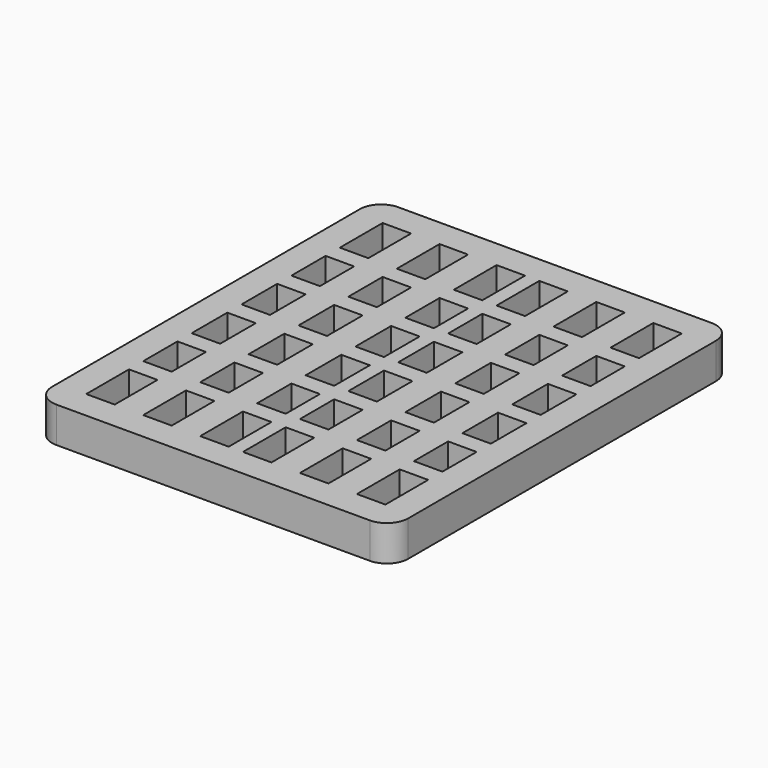
from build123d import *

# Parameters (mm, degrees)
F1_DEPTH = 5
F0_W     = 4
F0_H     = 7.5
F0_H_2   = 6.25
F0_H_3   = 6
F0_W_2   = 2
F0_H_4   = 2.5
F2_DEPTH = 5


# Not quite as in the source:
# - a feature names something its author has since deleted; it is built from what else it names


with BuildPart() as f1:
    # F0 (on Top) → F1 (new body)
    with BuildSketch(Plane.XY):
        with BuildLine():
            ThreePointArc((0, 3), (0.8786796564, 0.8786796564), (3, 0))
            Line((3, 0), (47, 0))
            ThreePointArc((47, 0), (49.1213203436, 0.8786796564), (50, 3))
            Line((50, 3), (50, 57))
            ThreePointArc((50, 57), (49.1213203436, 59.1213203436), (47, 60))
            Line((47, 60), (25, 60))
            Line((25, 60), (3, 60))
            ThreePointArc((3, 60), (0.8786796564, 59.1213203436), (0, 57))
            Line((0, 57), (0, 3))
        make_face()
        Polygon((24, 56), (25, 56), (26, 56), (30, 56), (34, 56), (38, 56), (42, 56), (46, 56), (46, 48.5), (46, 46), (46, 40), (46, 37.5), (46, 31.25), (46, 28.75), (46, 22.5), (46, 20), (46, 14), (46, 11.5), (46, 4), (42, 4), (38, 4), (34, 4), (30, 4), (26, 4), (24, 4), (20, 4), (16, 4), (12, 4), (8, 4), (4, 4), (4, 11.5), (4, 14), (4, 20), (4, 22.5), (4, 28.75), (4, 31.25), (4, 37.5), (4, 40), (4, 46), (4, 48.5), (4, 56), (8, 56), (12, 56), (16, 56), (20, 56), align=None, mode=Mode.SUBTRACT)
    extrude(amount=F1_DEPTH)

    # F0 (on Top) → F2 (join)
    with BuildSketch(Plane.XY):
        with BuildLine():
            ThreePointArc((0, 3), (0.8786796564, 0.8786796564), (3, 0))
            Line((3, 0), (47, 0))
            ThreePointArc((47, 0), (49.1213203436, 0.8786796564), (50, 3))
            Line((50, 3), (50, 57))
            ThreePointArc((50, 57), (49.1213203436, 59.1213203436), (47, 60))
            Line((47, 60), (25, 60))
            Line((25, 60), (3, 60))
            ThreePointArc((3, 60), (0.8786796564, 59.1213203436), (0, 57))
            Line((0, 57), (0, 3))
        make_face()
        Polygon((24, 56), (25, 56), (26, 56), (30, 56), (34, 56), (38, 56), (42, 56), (46, 56), (46, 48.5), (46, 46), (46, 40), (46, 37.5), (46, 31.25), (46, 28.75), (46, 22.5), (46, 20), (46, 14), (46, 11.5), (46, 4), (42, 4), (38, 4), (34, 4), (30, 4), (26, 4), (24, 4), (20, 4), (16, 4), (12, 4), (8, 4), (4, 4), (4, 11.5), (4, 14), (4, 20), (4, 22.5), (4, 28.75), (4, 31.25), (4, 37.5), (4, 40), (4, 46), (4, 48.5), (4, 56), (8, 56), (12, 56), (16, 56), (20, 56), align=None, mode=Mode.SUBTRACT)
        with Locations((18, 52.25)):
            Rectangle(F0_W, F0_H)
        with Locations((32, 52.25)):
            Rectangle(F0_W, F0_H)
        with Locations((10, 52.25)):
            Rectangle(F0_W, F0_H)
        with Locations((40, 52.25)):
            Rectangle(F0_W, F0_H)
        with Locations((18, 7.75)):
            Rectangle(F0_W, F0_H)
        with Locations((32, 7.75)):
            Rectangle(F0_W, F0_H)
        with Locations((10, 7.75)):
            Rectangle(F0_W, F0_H)
        with Locations((40, 7.75)):
            Rectangle(F0_W, F0_H)
        with Locations((18, 34.375)):
            Rectangle(F0_W, F0_H_2)
        with Locations((32, 34.375)):
            Rectangle(F0_W, F0_H_2)
        with Locations((10, 34.375)):
            Rectangle(F0_W, F0_H_2)
        with Locations((18, 25.625)):
            Rectangle(F0_W, F0_H_2)
        with Locations((40, 34.375)):
            Rectangle(F0_W, F0_H_2)
        with Locations((32, 25.625)):
            Rectangle(F0_W, F0_H_2)
        with Locations((10, 25.625)):
            Rectangle(F0_W, F0_H_2)
        with Locations((40, 25.625)):
            Rectangle(F0_W, F0_H_2)
        with Locations((18, 43)):
            Rectangle(F0_W, F0_H_3)
        with Locations((32, 43)):
            Rectangle(F0_W, F0_H_3)
        with Locations((10, 43)):
            Rectangle(F0_W, F0_H_3)
        with Locations((40, 43)):
            Rectangle(F0_W, F0_H_3)
        with Locations((18, 17)):
            Rectangle(F0_W, F0_H_3)
        with Locations((32, 17)):
            Rectangle(F0_W, F0_H_3)
        with Locations((10, 17)):
            Rectangle(F0_W, F0_H_3)
        with Locations((40, 17)):
            Rectangle(F0_W, F0_H_3)
        Polygon((26, 56), (25, 56), (24, 56), (24, 48.5), (26, 48.5), align=None)
        with Locations((25, 7.75)):
            Rectangle(F0_W_2, F0_H)
        with Locations((25, 34.375)):
            Rectangle(F0_W_2, F0_H_2)
        with Locations((25, 25.625)):
            Rectangle(F0_W_2, F0_H_2)
        with Locations((25, 43)):
            Rectangle(F0_W_2, F0_H_3)
        with Locations((25, 17)):
            Rectangle(F0_W_2, F0_H_3)
        with Locations((22, 47.25)):
            Rectangle(F0_W, F0_H_4)
        with Locations((28, 47.25)):
            Rectangle(F0_W, F0_H_4)
        with Locations((18, 47.25)):
            Rectangle(F0_W, F0_H_4)
        with Locations((32, 47.25)):
            Rectangle(F0_W, F0_H_4)
        with Locations((14, 47.25)):
            Rectangle(F0_W, F0_H_4)
        with Locations((22, 38.75)):
            Rectangle(F0_W, F0_H_4)
        with Locations((36, 47.25)):
            Rectangle(F0_W, F0_H_4)
        with Locations((28, 38.75)):
            Rectangle(F0_W, F0_H_4)
        with Locations((10, 47.25)):
            Rectangle(F0_W, F0_H_4)
        with Locations((18, 38.75)):
            Rectangle(F0_W, F0_H_4)
        with Locations((40, 47.25)):
            Rectangle(F0_W, F0_H_4)
        with Locations((32, 38.75)):
            Rectangle(F0_W, F0_H_4)
        with Locations((6, 47.25)):
            Rectangle(F0_W, F0_H_4)
        with Locations((14, 38.75)):
            Rectangle(F0_W, F0_H_4)
        with Locations((22, 30)):
            Rectangle(F0_W, F0_H_4)
        with Locations((44, 47.25)):
            Rectangle(F0_W, F0_H_4)
        with Locations((36, 38.75)):
            Rectangle(F0_W, F0_H_4)
        with Locations((28, 30)):
            Rectangle(F0_W, F0_H_4)
        with Locations((10, 38.75)):
            Rectangle(F0_W, F0_H_4)
        with Locations((18, 30)):
            Rectangle(F0_W, F0_H_4)
        with Locations((40, 38.75)):
            Rectangle(F0_W, F0_H_4)
        with Locations((32, 30)):
            Rectangle(F0_W, F0_H_4)
        with Locations((6, 38.75)):
            Rectangle(F0_W, F0_H_4)
        with Locations((14, 30)):
            Rectangle(F0_W, F0_H_4)
        with Locations((22, 21.25)):
            Rectangle(F0_W, F0_H_4)
        with Locations((44, 38.75)):
            Rectangle(F0_W, F0_H_4)
        with Locations((36, 30)):
            Rectangle(F0_W, F0_H_4)
        with Locations((28, 21.25)):
            Rectangle(F0_W, F0_H_4)
        with Locations((10, 30)):
            Rectangle(F0_W, F0_H_4)
        with Locations((18, 21.25)):
            Rectangle(F0_W, F0_H_4)
        with Locations((40, 30)):
            Rectangle(F0_W, F0_H_4)
        with Locations((32, 21.25)):
            Rectangle(F0_W, F0_H_4)
        with Locations((6, 30)):
            Rectangle(F0_W, F0_H_4)
        with Locations((14, 21.25)):
            Rectangle(F0_W, F0_H_4)
        with Locations((22, 12.75)):
            Rectangle(F0_W, F0_H_4)
        with Locations((44, 30)):
            Rectangle(F0_W, F0_H_4)
        with Locations((36, 21.25)):
            Rectangle(F0_W, F0_H_4)
        with Locations((28, 12.75)):
            Rectangle(F0_W, F0_H_4)
        with Locations((10, 21.25)):
            Rectangle(F0_W, F0_H_4)
        with Locations((18, 12.75)):
            Rectangle(F0_W, F0_H_4)
        with Locations((40, 21.25)):
            Rectangle(F0_W, F0_H_4)
        with Locations((32, 12.75)):
            Rectangle(F0_W, F0_H_4)
        with Locations((6, 21.25)):
            Rectangle(F0_W, F0_H_4)
        with Locations((14, 12.75)):
            Rectangle(F0_W, F0_H_4)
        with Locations((44, 21.25)):
            Rectangle(F0_W, F0_H_4)
        with Locations((36, 12.75)):
            Rectangle(F0_W, F0_H_4)
        with Locations((10, 12.75)):
            Rectangle(F0_W, F0_H_4)
        with Locations((40, 12.75)):
            Rectangle(F0_W, F0_H_4)
        with Locations((6, 12.75)):
            Rectangle(F0_W, F0_H_4)
        with Locations((44, 12.75)):
            Rectangle(F0_W, F0_H_4)
        with Locations((25, 47.25)):
            Rectangle(F0_W_2, F0_H_4)
        with Locations((25, 38.75)):
            Rectangle(F0_W_2, F0_H_4)
        with Locations((25, 30)):
            Rectangle(F0_W_2, F0_H_4)
        with Locations((25, 21.25)):
            Rectangle(F0_W_2, F0_H_4)
        with Locations((25, 12.75)):
            Rectangle(F0_W_2, F0_H_4)
    extrude(amount=F2_DEPTH)


solid = f1.part
